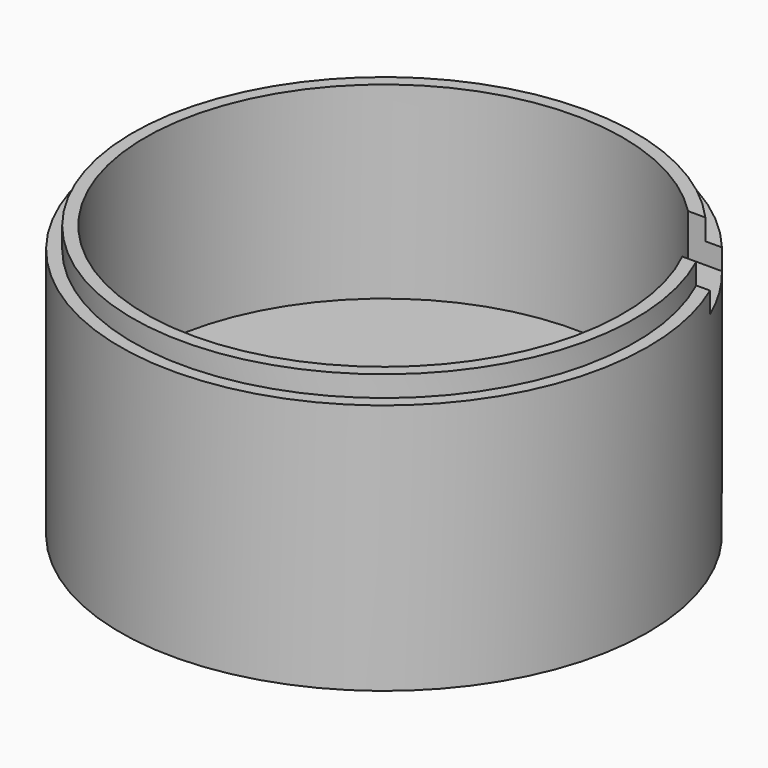
from build123d import *

# Parameters (mm, degrees)
F0_R      = 63
F0_R_2    = 60
F2_DEPTH  = 60
F1_R      = 60
F1_R_2    = 57
F3_DEPTH  = 65
F4_R      = 57
F5_DEPTH  = 60
F7_R      = 57
F8_DEPTH  = 40
F9_W      = 15
F9_H      = 10
F10_DEPTH = 279.5
F11_DEPTH = 71.5
F13_R     = 63
F14_DEPTH = 20
F15_W     = 86
F15_H     = 41
F16_DEPTH = 15
F17_W     = 27.3
F17_H     = 13
F18_DEPTH = 53
F20_DEPTH = 25


# Not quite as in the source:
# - a feature names something its author has since deleted; it is built from what else it names


with BuildPart() as f2:
    # F0 (on Top) → F2 (new body)
    with BuildSketch(Plane.XY):
        Circle(F0_R)
        Circle(F0_R_2, mode=Mode.SUBTRACT)
    extrude(amount=F2_DEPTH)

    # F1 (on Top) → F3 (join)
    with BuildSketch(Plane.XY):
        Circle(F1_R)
        Circle(F1_R_2, mode=Mode.SUBTRACT)
    extrude(amount=F3_DEPTH)

    # F4 (on Top) → F5 (join)
    with BuildSketch(Plane.XY):
        Circle(F4_R)
    extrude(amount=F5_DEPTH)

    # F7 (on offset) → F8 (cut)
    with BuildSketch(Plane.XY.offset(45)):
        Circle(F7_R)
    extrude(amount=-F8_DEPTH, mode=Mode.SUBTRACT)

    # F9 (on Right) → F10 (cut)
    with BuildSketch(Plane.YZ):
        with Locations((32.5, 60)):
            Rectangle(F9_W, F9_H)
    extrude(amount=F10_DEPTH, mode=Mode.SUBTRACT)

    # F1 (on Top) → F11 (cut)
    with BuildSketch(Plane.XY):
        Circle(F1_R_2)
    extrude(amount=F11_DEPTH, mode=Mode.SUBTRACT)

    # F13 (on Top) → F14 (join)
    with BuildSketch(Plane.XY):
        Circle(F13_R)
    extrude(amount=F14_DEPTH)

    # F15 (on Top) → F16 (cut)
    with BuildSketch(Plane.XY):
        Rectangle(F15_W, F15_H)
    extrude(amount=F16_DEPTH, mode=Mode.SUBTRACT)

    # F17 (on Right) → F18 (cut)
    with BuildSketch(Plane.YZ):
        with Locations((6.82, 8.5)):
            Rectangle(F17_W, F17_H)
    extrude(amount=F18_DEPTH, mode=Mode.SUBTRACT)

    # F19 (on offset) → F20 (cut)
    with BuildSketch(Plane.XY.offset(15)):
        Polygon((43, 20.47), (43, 0), (43, -6.83), (53, -6.83), (53, 20.47), align=None)
    extrude(amount=F20_DEPTH, mode=Mode.SUBTRACT)


solid = f2.part
